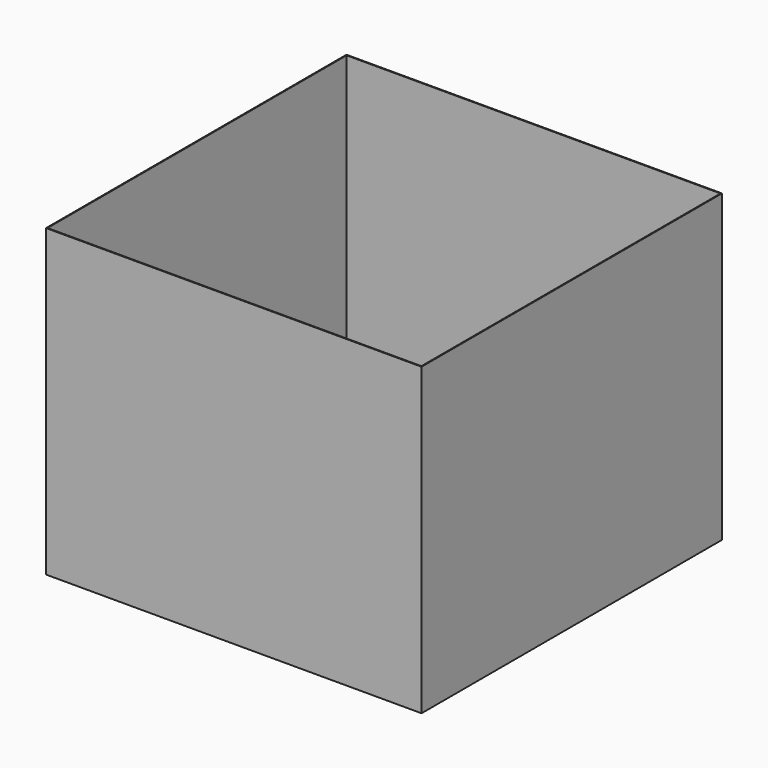
from build123d import *

# Parameters (mm, degrees)
F0_W     = 1219.2
F0_H     = 1219.2
F1_DEPTH = 990.6
F2_T     = -2.54


# Not quite as in the source:
# - the program builds the solid bodies; features that only make, move or delete a surface that nothing else refers to are left out


with BuildPart() as f1:
    # F0 (on Top) → F1 (new body)
    with BuildSketch(Plane.XY):
        Rectangle(F0_W, F0_H)
    extrude(amount=F1_DEPTH)

    # F2
    f2_openings = [f1.faces().sort_by_distance(p)[0] for p in [
        (0, 0, 990.6),
    ]]
    offset(amount=F2_T, openings=f2_openings)


solid = f1.part
